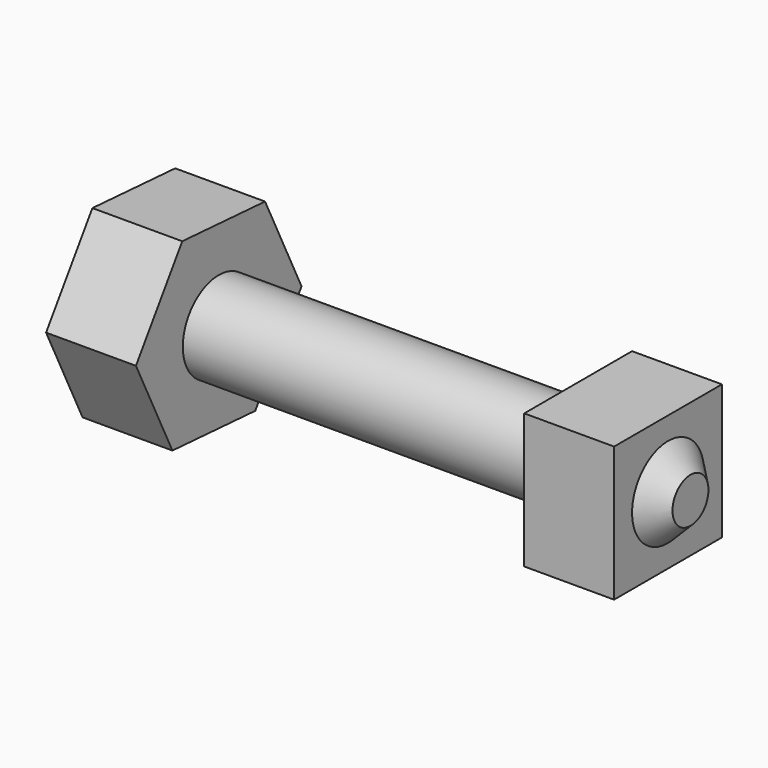
from build123d import *

# Parameters (mm, degrees)
F0_R     = 5
F1_DEPTH = 50
F3_DEPTH = 10
F4_W     = 15
F4_H     = 15
F4_R     = 5
F5_DEPTH = 10
F6_R     = 5
F7_DEPTH = 2.5
F8_SIZE  = 2.49999


# Not quite as in the source:
# - a fillet or chamfer is up to 0.001 mm smaller than in the source, because OpenCascade refuses the exact size


with BuildPart() as f1:
    # F0 (on Right) → F1 (new body)
    with BuildSketch(Plane.YZ):
        Circle(F0_R)
    extrude(amount=F1_DEPTH)

    # F2 (on face) → F3 (join)
    with BuildSketch(Plane(origin=(0, 0, 0), x_dir=(0, -1, 0), z_dir=(-1, 0, 0))):
        Polygon((11.5200223266, 0.788935313), (5.0767731403, 10.3710996435), (-6.4432491863, 9.5821643305), (-11.5200223266, -0.788935313), (-5.0767731403, -10.3710996435), (6.4432491863, -9.5821643305), align=None)
    extrude(amount=F3_DEPTH)

    # F4 (on face) → F5 (join)
    with BuildSketch(Plane.YZ.offset(50)):
        Rectangle(F4_W, F4_H)
        Circle(F4_R, mode=Mode.SUBTRACT)
    extrude(amount=-F5_DEPTH)

    # F6 (on face) → F7 (join)
    with BuildSketch(Plane.YZ.offset(50)):
        Circle(F6_R)
    extrude(amount=F7_DEPTH)

    # F8 (size 2.5 in the source; OpenCascade refuses exactly that, so slightly less here)
    f8_edges = [f1.edges().sort_by_distance(p)[0] for p in [
        (52.5, -5, 0),
    ]]
    chamfer(f8_edges, length=F8_SIZE)


solid = f1.part
